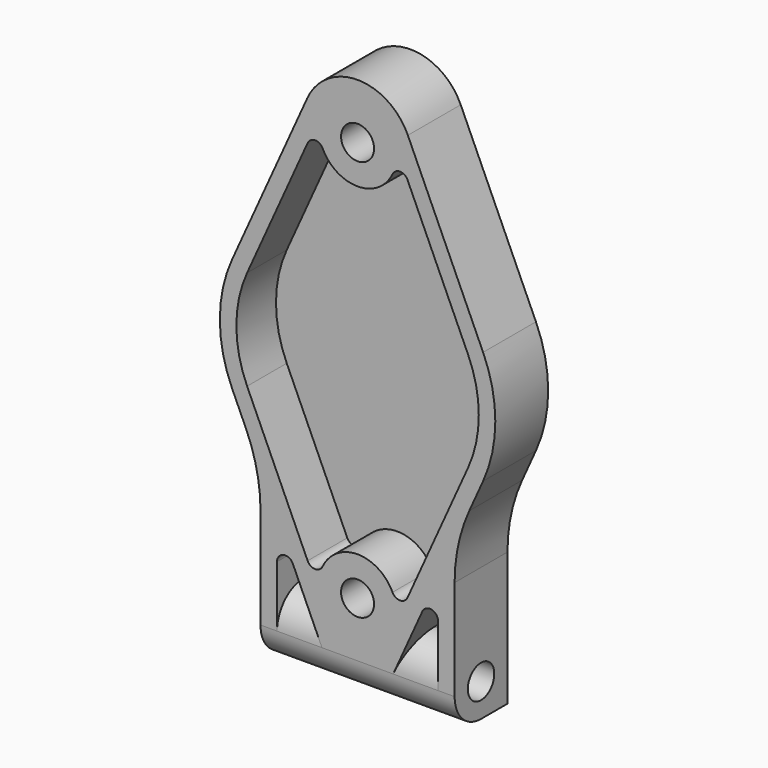
from build123d import *

# Parameters (mm, degrees)
F0_R     = 2
F1_DEPTH = 8
F2_DEPTH = 2
F3_R     = 20
F4_R     = 1
F6_D     = 4
F7_R     = 3.99999


# Not quite as in the source:
# - a fillet or chamfer is up to 0.001 mm smaller than in the source, because OpenCascade refuses the exact size
# - a feature names something its author has since deleted; it is built from what else it names


with BuildPart() as f1:
    # F0 (on Front) → F1 (new body)
    with BuildSketch(Plane.XZ):
        with BuildLine():
            Line((15.1970139668, 6.8636525628), (6.0880650012, 27.0320429916))
            ThreePointArc((6.0880650012, 27.0320429916), (0, 30.9626), (-6.0880650012, 27.0320429916))
            Line((-6.0880650012, 27.0320429916), (-15.1970139668, 6.8636525628))
            ThreePointArc((-15.1970139668, 6.8636525628), (-16.6751, 0), (-15.1970139668, -6.8636525628))
            Line((-15.1970139668, -6.8636525628), (-11.75, -14.4957870449))
            Line((-11.75, -14.4957870449), (-9.75, -18.9240455641))
            Line((-9.75, -18.9240455641), (-6.1194285683, -26.9626))
            Line((-6.1194285683, -26.9626), (6.1194285683, -26.9626))
            Line((6.1194285683, -26.9626), (9.75, -18.9240455641))
            Line((9.75, -18.9240455641), (11.75, -14.4957870449))
            Line((11.75, -14.4957870449), (15.1970139668, -6.8636525628))
            ThreePointArc((15.1970139668, -6.8636525628), (16.6751, 0), (15.1970139668, 6.8636525628))
        make_face()
        with Locations((0, -24.2824)):
            Circle(F0_R, mode=Mode.SUBTRACT)
        with BuildLine():
            Line((-13.3742945868, 6.0404308054), (-6.0462846285, 22.2655920687))
            ThreePointArc((-6.0462846285, 22.2655920687), (-5.1436901116, 22.8539427752), (-4.2309206889, 22.2815046593))
            ThreePointArc((-4.2309206889, 22.2815046593), (0, 19.6022), (4.2309206889, 22.2815046593))
            ThreePointArc((4.2309206889, 22.2815046593), (5.1436901116, 22.8539427752), (6.0462846285, 22.2655920687))
            Line((6.0462846285, 22.2655920687), (13.3742945868, 6.0404308054))
            ThreePointArc((13.3742945868, 6.0404308054), (14.6751, 0), (13.3742945868, -6.0404308054))
            Line((13.3742945868, -6.0404308054), (6.0462846285, -22.2655920687))
            ThreePointArc((6.0462846285, -22.2655920687), (5.1436901116, -22.8539427752), (4.2309206889, -22.2815046593))
            ThreePointArc((4.2309206889, -22.2815046593), (0, -19.6022), (-4.2309206889, -22.2815046593))
            ThreePointArc((-4.2309206889, -22.2815046593), (-5.1436901116, -22.8539427752), (-6.0462846285, -22.2655920687))
            Line((-6.0462846285, -22.2655920687), (-13.3742945868, -6.0404308054))
            ThreePointArc((-13.3742945868, -6.0404308054), (-14.6751, 0), (-13.3742945868, 6.0404308054))
        make_face(mode=Mode.SUBTRACT)
        with Locations((0, 24.2824)):
            Circle(F0_R, mode=Mode.SUBTRACT)
        Polygon((11.75, -34.9626), (11.75, -14.4957870449), (9.75, -18.9240455641), (9.75, -26.9626), (6.1194285683, -26.9626), (-6.1194285683, -26.9626), (-9.75, -26.9626), (-9.75, -18.9240455641), (-11.75, -14.4957870449), (-11.75, -34.9626), align=None)
    extrude(amount=F1_DEPTH)

    # F0 (on Front) → F2 (join)
    with BuildSketch(Plane.XZ):
        with BuildLine():
            ThreePointArc((-4.2309206889, 22.2815046593), (-5.1436901116, 22.8539427752), (-6.0462846285, 22.2655920687))
            Line((-6.0462846285, 22.2655920687), (-13.3742945868, 6.0404308054))
            ThreePointArc((-13.3742945868, 6.0404308054), (-14.6751, 0), (-13.3742945868, -6.0404308054))
            Line((-13.3742945868, -6.0404308054), (-6.0462846285, -22.2655920687))
            ThreePointArc((-6.0462846285, -22.2655920687), (-5.1436901116, -22.8539427752), (-4.2309206889, -22.2815046593))
            ThreePointArc((-4.2309206889, -22.2815046593), (0, -19.6022), (4.2309206889, -22.2815046593))
            ThreePointArc((4.2309206889, -22.2815046593), (5.1436901116, -22.8539427752), (6.0462846285, -22.2655920687))
            Line((6.0462846285, -22.2655920687), (13.3742945868, -6.0404308054))
            ThreePointArc((13.3742945868, -6.0404308054), (14.6751, 0), (13.3742945868, 6.0404308054))
            Line((13.3742945868, 6.0404308054), (6.0462846285, 22.2655920687))
            ThreePointArc((6.0462846285, 22.2655920687), (5.1436901116, 22.8539427752), (4.2309206889, 22.2815046593))
            ThreePointArc((4.2309206889, 22.2815046593), (0, 19.6022), (-4.2309206889, 22.2815046593))
        make_face()
        Polygon((11.75, -34.9626), (11.75, -14.4957870449), (9.75, -18.9240455641), (9.75, -26.9626), (6.1194285683, -26.9626), (-6.1194285683, -26.9626), (-9.75, -26.9626), (-9.75, -18.9240455641), (-11.75, -14.4957870449), (-11.75, -34.9626), align=None)
        Polygon((-6.1194285683, -26.9626), (-9.75, -18.9240455641), (-9.75, -26.9626), align=None)
        Polygon((9.75, -26.9626), (9.75, -18.9240455641), (6.1194285683, -26.9626), align=None)
    extrude(amount=F2_DEPTH)

    # F3
    f3_edges = [f1.edges().sort_by_distance(p)[0] for p in [
        (11.75, -4, -14.495787),
        (-11.75, -4, -14.495787),
    ]]
    fillet(f3_edges, radius=F3_R)

    # F4
    f4_edges = [f1.edges().sort_by_distance(p)[0] for p in [
        (9.75, -5, -18.924046),
        (-9.75, -5, -18.924046),
    ]]
    fillet(f4_edges, radius=F4_R)

    # F6 (through all)
    with Locations(Plane.YZ.offset(11.75)):
        with Locations((-4, -30.9626)):
            Hole(F6_D / 2)

    # F7 (radius 4 in the source; OpenCascade refuses exactly that, so slightly less here)
    f7_edges = [f1.edges().sort_by_distance(p)[0] for p in [
        (0, -8, -34.9626),
        (7.934714, -8, -26.9626),
        (-7.934714, -8, -26.9626),
    ]]
    fillet(f7_edges, radius=F7_R)


solid = f1.part
